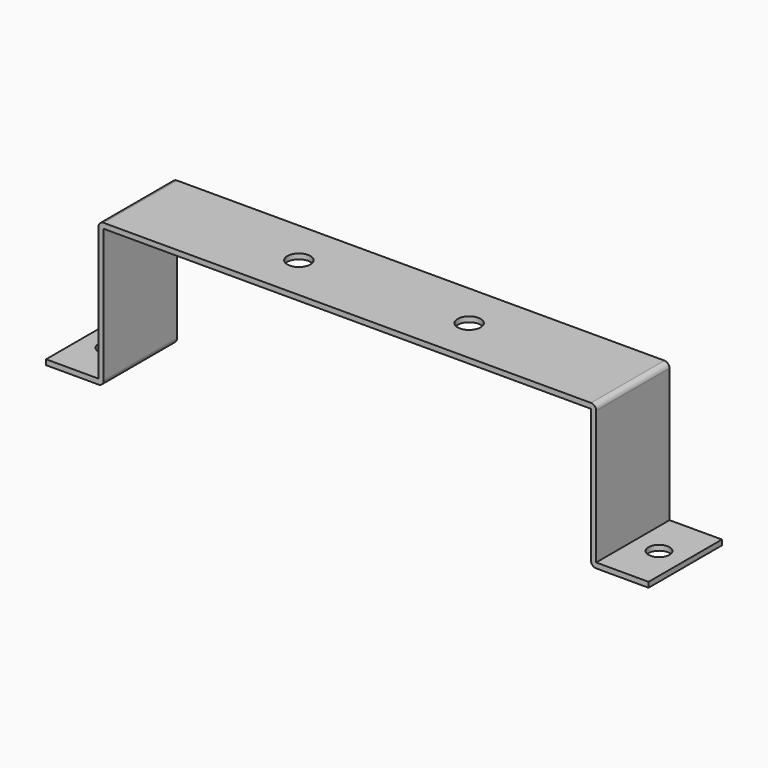
from build123d import *

# Parameters (mm, degrees)
F1_DEPTH = 17.5
F2_R     = 4
F3_DEPTH = 25
F4_R     = 4.4
F5_DEPTH = 25
F6_R     = 2


# Not quite as in the source:
# - a feature names something its author has since deleted; it is built from what else it names


with BuildPart() as f1:
    # F0 (on Front) → F1 (new body, symmetric)
    with BuildSketch(Plane.XZ):
        Polygon((95, -38), (95, 15), (-95, 15), (-95, -38), (-115, -38), (-115, -40), (-93, -40), (-93, 13), (93, 13), (93, -40), (115, -40), (115, -38), align=None)
    extrude(amount=F1_DEPTH, both=True)

    # F2 (on face) → F3 (cut)
    with BuildSketch(Plane.XY.offset(-38)):
        with Locations((-105, 0)):
            Circle(F2_R)
        with Locations((105, 0)):
            Circle(F2_R)
    extrude(amount=-F3_DEPTH, mode=Mode.SUBTRACT)

    # F4 (on face) → F5 (cut)
    with BuildSketch(Plane.XY.offset(15)):
        with Locations((-32.5, 0)):
            Circle(F4_R)
        with Locations((32.5, 0)):
            Circle(F4_R)
    extrude(amount=-F5_DEPTH, mode=Mode.SUBTRACT)

    # F6
    f6_edges = [f1.edges().sort_by_distance(p)[0] for p in [
        (95, 0, 15),
        (-95, 0, 15),
        (-93, 0, -40),
        (93, 0, -40),
    ]]
    fillet(f6_edges, radius=F6_R)


solid = f1.part
